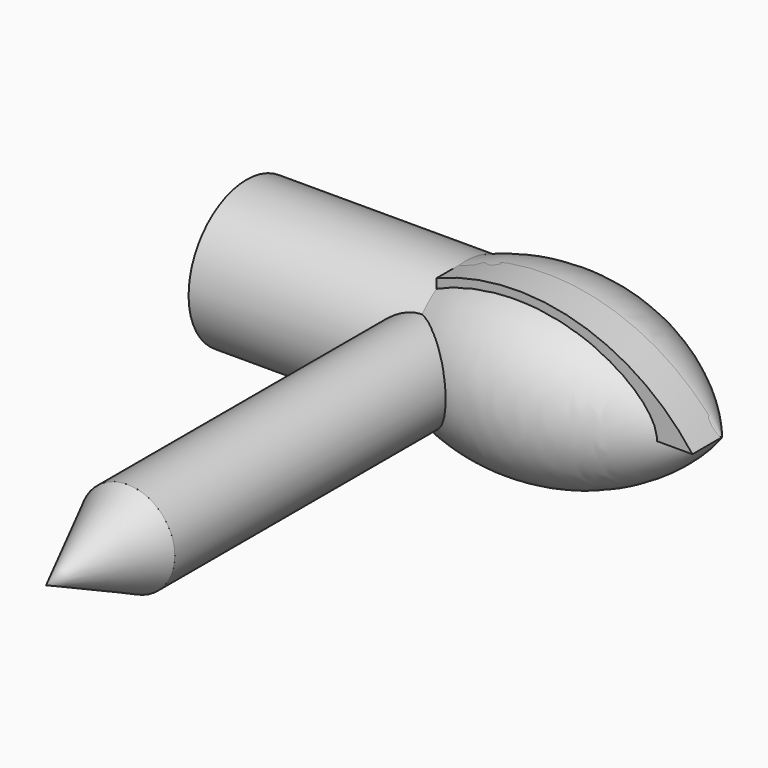
from build123d import *

# Parameters (mm, degrees)
F0_R     = 16.51
F0_R_2   = 12.7
F1_DEPTH = 147.32
F2_R     = 16.51
F7_DEPTH = 12.7


# Not quite as in the source:
# - an extrude whose draft closes it to a point is written as a loft to that point


with BuildPart() as f1:
    # F0 (on Front) → F1 (new body)
    with BuildSketch(Plane.XZ):
        Circle(F0_R)
        Circle(F0_R_2, mode=Mode.SUBTRACT)
    extrude(amount=F1_DEPTH)

    # F2 (on face) → F3 section 0
    with BuildSketch(Plane.XZ.offset(147.32), mode=Mode.PRIVATE) as f3_s0:
        Circle(F2_R)
    loft([f3_s0.sketch, Vertex(0, -182.7258092576, 0)], ruled=True)


with BuildPart() as f5:
    # F4 (on Front) → F5 (revolve)
    with BuildSketch(Plane.XZ):
        with BuildLine():
            Line((61.5253970027, 0), (89.1491068253, 0))
            ThreePointArc((89.1491068253, 0), (48.7342366617, 27.3129928395), (0, 25.2308100462))
            Line((0, 25.2308100462), (-76.3670504093, 25.2308100462))
            Line((-76.3670504093, 25.2308100462), (-76.3670504093, 15.7861206681))
            Line((-76.3670504093, 15.7861206681), (0, 15.7861206681))
            ThreePointArc((0, 15.7861206681), (32.4318819895, 14.3985963638), (61.5253970027, 0))
        make_face()
    revolve(axis=Axis((75.337251914, 0, 0), (-1, 0, 0)))


with BuildPart() as f7:
    # F6 (on Front) → F7 (new body)
    with BuildSketch(Plane.XZ):
        with BuildLine():
            ThreePointArc((89.0533104539, 0), (48.7563256153, 27.5615607886), (0, 25.0501204282))
            Line((0, 25.0501204282), (0, 15.8704593778))
            ThreePointArc((0, 15.8704593778), (32.405246833, 14.3232478343), (61.5143254399, 0))
            Line((61.5143254399, 0), (89.0533104539, 0))
        make_face()
    extrude(amount=F7_DEPTH)


solid = Compound([f1.part, f5.part, f7.part])
